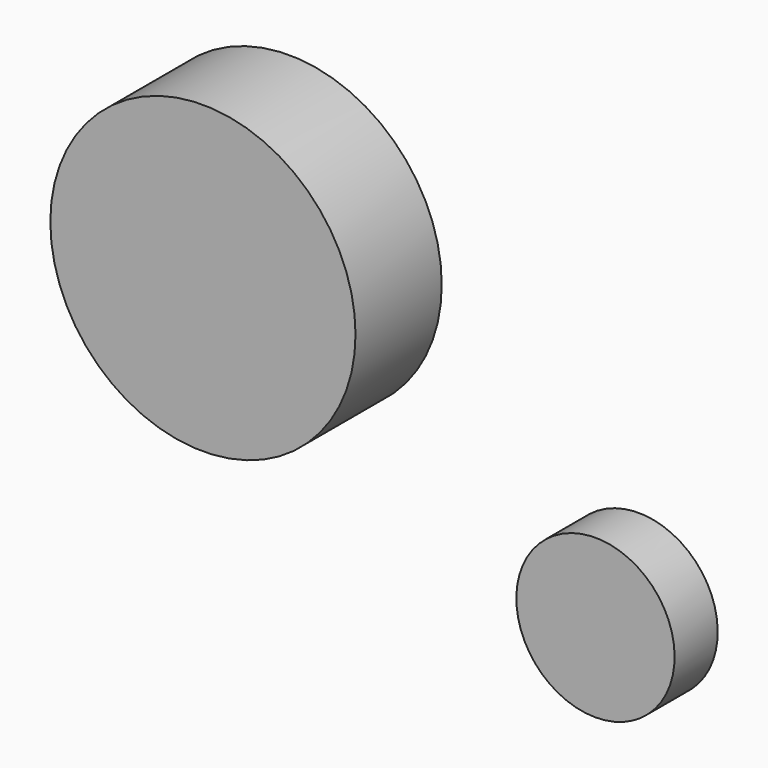
from build123d import *

# Parameters (mm, degrees)
F1_DEPTH = 25.4
F2_DEPTH = 12.7


with BuildPart() as f1:
    # F0 (on Front) → F1 (new body)
    with BuildSketch(Plane.XZ):
        with BuildLine():
            ThreePointArc((-13.128761544, -33.488874266), (20.2684777915, -29.7162899316), (35.9703917032, 0))
            ThreePointArc((35.9703917032, 0), (20.2684777915, 29.7162899316), (-13.128761544, 33.488874266))
            ThreePointArc((-13.128761544, 33.488874266), (-35.9703917032, 0), (-13.128761544, -33.488874266))
        make_face()
    extrude(amount=F1_DEPTH)


with BuildPart() as f2:
    # F0 (on Front) → F2 (new body)
    with BuildSketch(Plane.XZ):
        with BuildLine():
            ThreePointArc((101.021352664, -50.8948202871), (71.8610828041, -35.4867042121), (75.5630787029, -68.2590493472))
            ThreePointArc((75.5630787029, -68.2590493472), (92.8797942312, -66.3029363622), (101.021352664, -50.8948202871))
        make_face()
    extrude(amount=F2_DEPTH)


solid = Compound([f1.part, f2.part])
